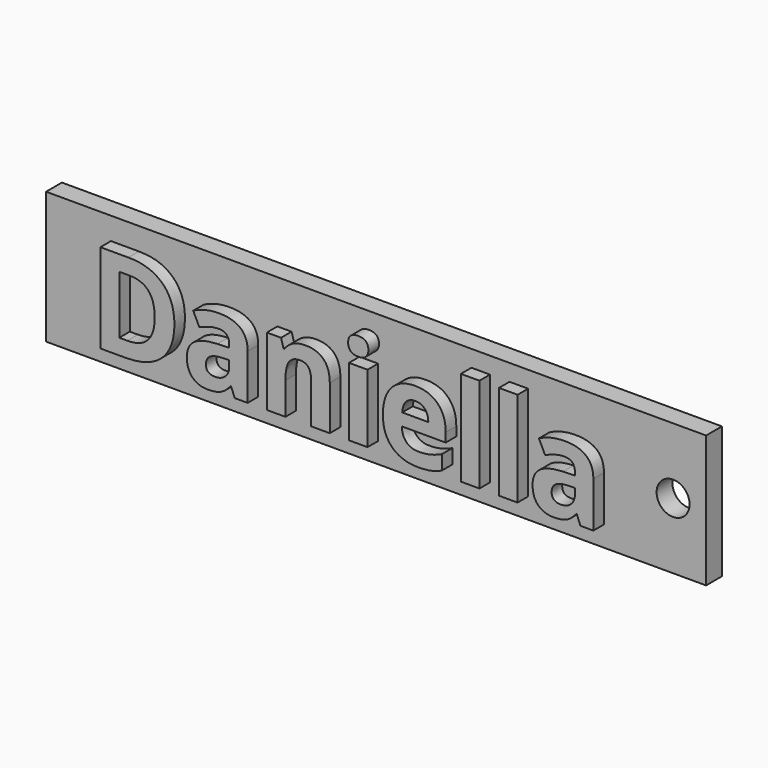
from build123d import *

# Parameters (mm, degrees)
F0_W         = 100
F0_H         = 20
F0_R         = 2.5
F1_DEPTH     = 3
F2_TEXT_SIZE = 18.9267887941
F3_DEPTH     = 5


# Not quite as in the source:
# - Text() gives the source's letters only with a copy of the font that has no kerning and outlines rounded to 1/6400 em; it was checked with that copy


with BuildPart() as f1:
    # F0 (on Front) → F1 (new body)
    with BuildSketch(Plane.XZ):
        with Locations((50, -10)):
            Rectangle(F0_W, F0_H)
        with Locations((95, -10)):
            Circle(F0_R, mode=Mode.SUBTRACT)
    extrude(amount=F1_DEPTH)

    # F2 (on Front) → F3 (join)
    with BuildSketch(Plane.XZ):
        with Locations((8.1239817664, -16.9030781835)):
            Text('Daniella', F2_TEXT_SIZE, font='Open Sans', font_style=FontStyle.BOLD, text_align=(TextAlign.LEFT, TextAlign.BOTTOM))
    extrude(amount=F3_DEPTH)


solid = f1.part
